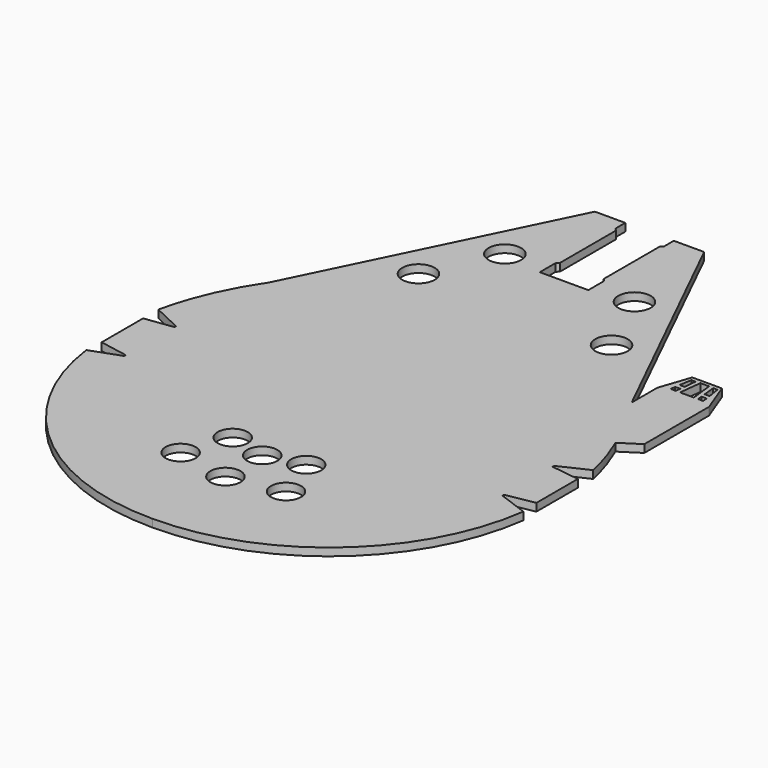
from build123d import *

# Parameters (mm, degrees)
F0_R     = 1.9381566851
F0_R_2   = 2.0917368597
F1_DEPTH = 1


# Not quite as in the source:
# - a feature names something its author has since deleted; it is built from what else it names


with BuildPart() as f1:
    # F0 (on Top) → F1 (new body)
    with BuildSketch(Plane.XY):
        with BuildLine():
            Line((3.1245559464, 26.2624721611), (-1.08e-08, 26.2624721611))
            Line((-1.08e-08, 26.2624721611), (-3.124555968, 26.2624721611))
            Line((-3.124555968, 26.2624721611), (-3.124555968, 28.8313598976))
            Line((-3.124555968, 28.8313598976), (-3.124555968, 38.4353779081))
            Line((-3.124555968, 38.4353779081), (-3.124555968, 40.0192436593))
            Line((-3.124555968, 40.0192436593), (-7.0351105106, 40.0192436593))
            Line((-7.0351105106, 40.0192436593), (-22.9566536529, 7.5476728616))
            add(Edge.make_bspline(
                [(-22.9566536529, 7.5476728616), (-25.3127067939, 4.1178797379), (-27.103694983, 0.0661364302), (-27.9845091561, -4.0443276364)],
                knots=[0, 0, 0, 0, 12.635418731, 12.635418731, 12.635418731, 12.635418731], degree=3))
            Line((-27.9845091561, -4.0443276364), (-24.3406626732, -5.7663835679))
            Line((-24.3406626732, -5.7663835679), (-24.3406626732, -6.0127781864))
            Line((-24.3406626732, -6.0127781864), (-27.9845091561, -6.501597853))
            Line((-27.9845091561, -6.501597853), (-27.9845091561, -13.1704901951))
            Line((-27.9845091561, -13.1704901951), (-24.3406626732, -13.83388813))
            Line((-24.3406626732, -13.83388813), (-24.3406626732, -14.0802827486))
            Line((-24.3406626732, -14.0802827486), (-28.1370117447, -15.4628727929))
            ThreePointArc((-28.1370117447, -15.4628727929), (-18.7026452725, -33.0246464869), (-0.0200514, -39.9804967013))
            ThreePointArc((-0.0200514, -39.9804967013), (-0.0100256971, -39.9804519319), (-1.08e-08, -39.9804036034))
            ThreePointArc((-1.08e-08, -39.9804036034), (18.6950876239, -33.0312342783), (28.1370117231, -15.4628727929))
            Line((28.1370117231, -15.4628727929), (24.3406626516, -14.0802827486))
            Line((24.3406626516, -14.0802827486), (24.3406626516, -13.8338881301))
            Line((24.3406626516, -13.8338881301), (27.9845091345, -13.1704901951))
            Line((27.9845091345, -13.1704901951), (27.9845091345, -6.501597853))
            Line((27.9845091345, -6.501597853), (24.3406626516, -6.0127781865))
            Line((24.3406626516, -6.0127781865), (24.3406626516, -5.7663835679))
            Line((24.3406626516, -5.7663835679), (27.9845091345, -4.0443276364))
            add(Edge.make_bspline(
                [(26.0221502825, 2.0106991689), (26.8752917045, 0.0540824437), (27.5438186439, -1.9877730517), (27.9845091345, -4.0443276364)],
                knots=[6.3136438899, 6.3136438899, 6.3136438899, 6.3136438899, 12.635418731, 12.635418731, 12.635418731, 12.635418731], degree=3))
            add(Edge.make_bspline(
                [(22.9566536312, 7.5476728616), (24.1339221361, 5.8338798437), (25.1701061555, 3.9647993294), (26.0221502825, 2.0106991689)],
                knots=[0, 0, 0, 0, 6.3136438899, 6.3136438899, 6.3136438899, 6.3136438899], degree=3))
            Line((22.9566536312, 7.5476728616), (21.8193497392, 9.8671744024))
            Line((21.8193497392, 9.8671744024), (7.035110489, 40.0192436593))
            Line((7.035110489, 40.0192436593), (3.1245559464, 40.0192436593))
            Line((3.1245559464, 40.0192436593), (3.1245559464, 38.4353779081))
            Line((3.1245559464, 38.4353779081), (3.1245559464, 28.8313598976))
            Line((3.1245559464, 28.8313598976), (3.1245559464, 26.2624721611))
        make_face()
        with Locations((-6.7846685267, -26.966459513)):
            Circle(F0_R, mode=Mode.SUBTRACT)
        with Locations((-1.08e-08, -28.2356044358)):
            Circle(F0_R, mode=Mode.SUBTRACT)
        with Locations((-4.7346279243, -21.1471724542)):
            Circle(F0_R, mode=Mode.SUBTRACT)
        with Locations((-1.08e-08, -22.3102177961)):
            Circle(F0_R, mode=Mode.SUBTRACT)
        with Locations((6.784668505, -26.966459513)):
            Circle(F0_R, mode=Mode.SUBTRACT)
        with Locations((4.7346279027, -21.1471724542)):
            Circle(F0_R, mode=Mode.SUBTRACT)
        with Locations((-12.4288502443, 18.366707164)):
            Circle(F0_R_2, mode=Mode.SUBTRACT)
        with Locations((-8.3437176479, 27.1654560115)):
            Circle(F0_R_2, mode=Mode.SUBTRACT)
        with Locations((12.4288502227, 18.366707164)):
            Circle(F0_R_2, mode=Mode.SUBTRACT)
        with Locations((8.3437176263, 27.1654560115)):
            Circle(F0_R_2, mode=Mode.SUBTRACT)
        with BuildLine():
            Line((21.8193497392, 14.0026268734), (21.8193497392, 9.8671744024))
            Line((21.8193497392, 9.8671744024), (22.9566536312, 7.5476728616))
            add(Edge.make_bspline(
                [(22.9566536312, 7.5476728616), (24.1339221361, 5.8338798437), (25.1701061555, 3.9647993294), (26.0221502825, 2.0106991689)],
                knots=[0, 0, 0, 0, 6.3136438899, 6.3136438899, 6.3136438899, 6.3136438899], degree=3))
            Line((26.0221502825, 2.0106991689), (28.4720553036, 3.5966005617))
            Line((28.4720553036, 3.5966005617), (28.4720553036, 14.0026268734))
            Line((28.4720553036, 14.0026268734), (26.9772648538, 17.9472138793))
            Line((26.9772648538, 17.9472138793), (23.1570666214, 17.9472138793))
            Line((23.1570666214, 17.9472138793), (21.8193497392, 14.0026268734))
        make_face()
        Polygon((23.0341097003, 14.6254569428), (23.103940836, 15.2695124223), (23.7673383417, 15.2695124223), (23.6930889239, 14.6254569428), align=None, mode=Mode.SUBTRACT)
        Polygon((27.2249650291, 14.6254569428), (26.5659858056, 14.6254569428), (26.4917363877, 15.2695124223), (27.1551338935, 15.2695124223), align=None, mode=Mode.SUBTRACT)
        Polygon((23.1912288972, 15.8630787924), (23.4530965144, 17.4342844956), (23.9942903911, 17.4342844956), (23.8371694774, 15.8630787924), align=None, mode=Mode.SUBTRACT)
        Polygon((24.238699366, 14.6254569428), (24.5689903023, 17.4904718284), (25.6900844272, 17.4904718284), (26.0203753635, 14.6254569428), align=None, mode=Mode.SUBTRACT)
        Polygon((27.0678458323, 15.8630787924), (26.4219052521, 15.8630787924), (26.2647843384, 17.4342844956), (26.8059782151, 17.4342844956), align=None, mode=Mode.SUBTRACT)
        Polygon((-3.124555968, 38.4353779081), (-3.124555968, 28.8313598976), (-2.8081914709, 29.1106844403), (-2.8081914709, 38.1560533654), align=None)
        Polygon((2.8081914492, 29.1106844403), (3.1245559464, 28.8313598976), (3.1245559464, 38.4353779081), (2.8081914492, 38.1560533654), align=None)
    extrude(amount=F1_DEPTH)


solid = f1.part
